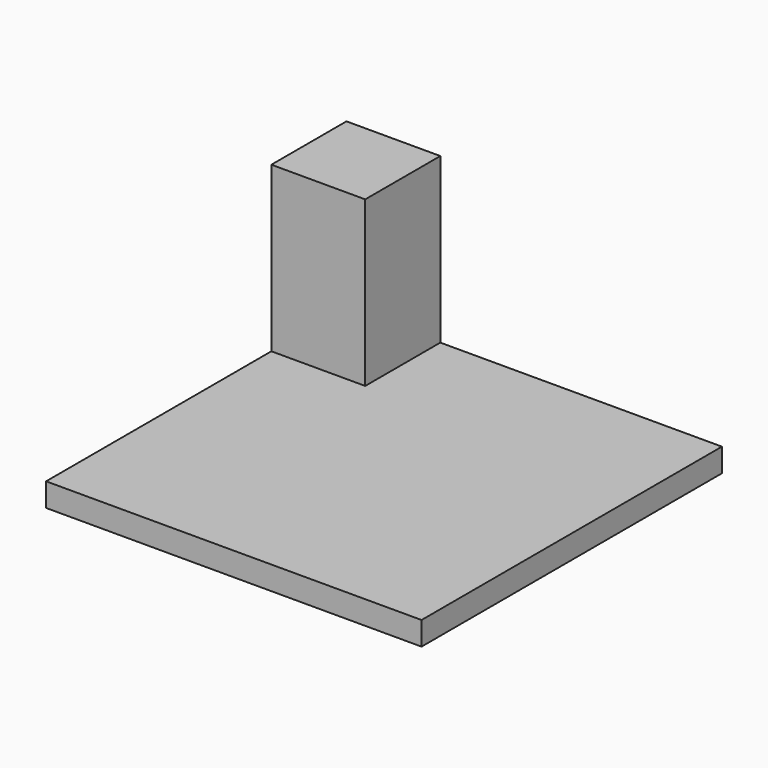
from build123d import *

# Parameters (mm, degrees)
F1_DEPTH = 1.5875
F0_W     = 6.35
F0_H     = 6.35
F2_DEPTH = 12.7


# Not quite as in the source:
# - a length typed as a fraction of an inch, garbled in the dataset ("3 / 203.2 mm" for 3/8 in), is restored


with BuildPart() as f1:
    # F0 (on Top) → F1 (new body)
    with BuildSketch(Plane.XY):
        Polygon((-12.7, -12.7), (12.7, -12.7), (12.7, 12.7), (-6.35, 12.7), (-6.35, 6.35), (-12.7, 6.35), align=None)
    extrude(amount=F1_DEPTH)

    # F0 (on Top) → F2 (join)
    with BuildSketch(Plane.XY):
        with Locations((-9.525, 9.525)):
            Rectangle(F0_W, F0_H)
    extrude(amount=F2_DEPTH)


solid = f1.part
